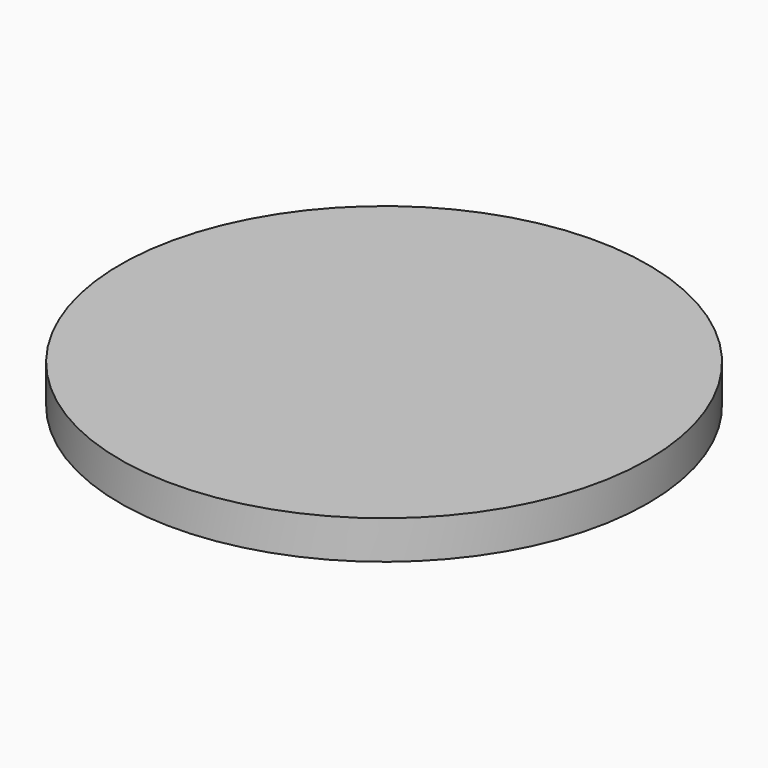
from build123d import *

# Parameters (mm, degrees)
F0_R     = 34.925
F5_DEPTH = 5.08


# Not quite as in the source:
# - the program builds the solid bodies; features that only make, move or delete a surface that nothing else refers to are left out


with BuildPart() as f5:
    # F0 (on Top) → F5 (new body)
    with BuildSketch(Plane.XY):
        Circle(F0_R)
    extrude(amount=-F5_DEPTH)


solid = f5.part
